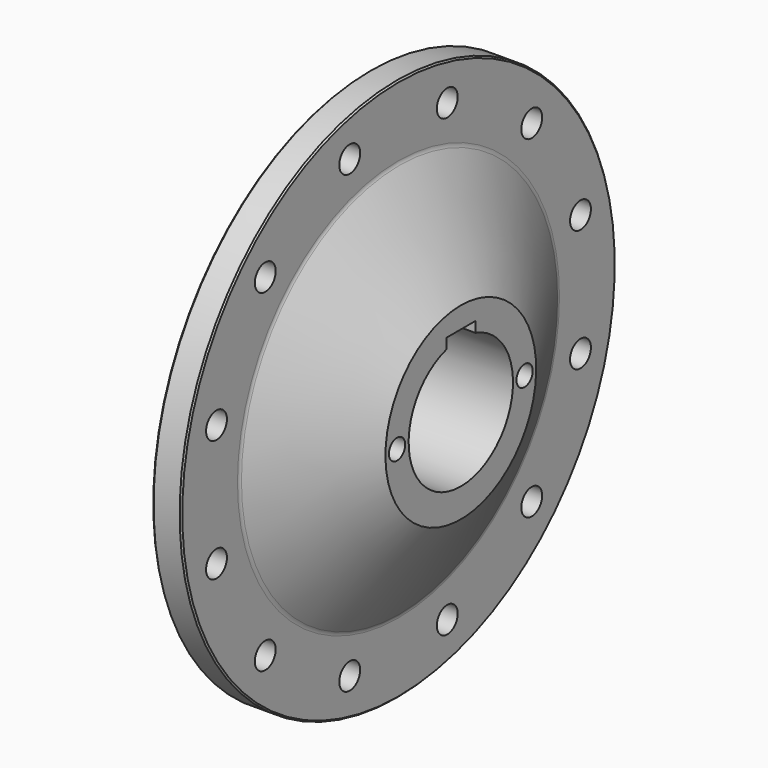
from build123d import *

# Parameters (mm, degrees)
F2_SIZE2         = 0.5358983849
F2_SIZE          = 2
F3_R             = 5
F4_SIZE          = 1
F5_R             = 2
F6_R             = 3
F8_D             = 14
F8_DEPTH         = 30
F8_TIP           = 4.2060243332
F9_W             = 25
F9_H             = 14
F10_DEPTH        = 133.001
F11_R            = 9
F12_DEPTH        = 25
F12_COPIES_COUNT = 12


# Not quite as in the source:
# - a pattern or mirror of a feature is missing from the dataset's text; its kind, count and spacing are read off the source's solid


with BuildPart() as f1:
    # F0 (on Front) → F1 (revolve)
    with BuildSketch(Plane.XZ):
        Polygon((0, 65), (0, 45), (133, 45), (133, 65), (90, 137.5), (90, 187.5), (70, 187.5), (70, 137.5), (60, 137.5), (60, 65), align=None)
    revolve(axis=Axis((87.7174822803, 0, 0), (1, 0, 0)))

    # F2
    f2_edges = [f1.edges().sort_by_distance(p)[0] for p in [
        (60, 0, -137.5),
    ]]
    chamfer(f2_edges, length=F2_SIZE, length2=F2_SIZE2)

    # F3
    f3_edges = [f1.edges().sort_by_distance(p)[0] for p in [
        (60, 0, -65),
        (90, 0, -137.5),
    ]]
    fillet(f3_edges, radius=F3_R)

    # F4
    f4_edges = [f1.edges().sort_by_distance(p)[0] for p in [
        (0, 0, -65),
        (70, 0, -187.5),
        (90, 0, -187.5),
    ]]
    chamfer(f4_edges, length=F4_SIZE)

    # F5
    f5_edges = [f1.edges().sort_by_distance(p)[0] for p in [
        (70, 0, -137.5),
    ]]
    fillet(f5_edges, radius=F5_R)

    # F6
    f6_edges = [f1.edges().sort_by_distance(p)[0] for p in [
        (0, 0, -45),
    ]]
    fillet(f6_edges, radius=F6_R)

    # F8
    with Locations(Plane.YZ.offset(133)):
        with Locations((55, 0), (-55, 0)):
            Hole(F8_D / 2, depth=F8_DEPTH)
            with Locations((0, 0, -(F8_DEPTH + F8_TIP / 2))):  # 118° drill point
                Cone(0, F8_D / 2, F8_TIP, mode=Mode.SUBTRACT)

    # F9 (on face) → F10 (cut, through all)
    with BuildSketch(Plane.YZ.offset(133)):
        with Locations((0, 43.4)):
            Rectangle(F9_W, F9_H)
    extrude(amount=-F10_DEPTH, mode=Mode.SUBTRACT)

    # F11 (on face) → F12 (cut)
    with BuildSketch(Plane(origin=(70, 0, 0), x_dir=(0, -1, 0), z_dir=(-1, 0, 0))):
        with Locations((156.962946772, 42.0580948292)):
            Circle(F11_R)
    f12 = extrude(amount=-F12_DEPTH, mode=Mode.SUBTRACT)

    # F12_copies: F12 ×12 about axis
    f12_copies_axis = Axis((0, 0, 0), (1, 0, 0))
    for i in range(1, F12_COPIES_COUNT):
        add(f12.rotate(f12_copies_axis, i * 360 / F12_COPIES_COUNT), mode=Mode.SUBTRACT)


solid = f1.part
